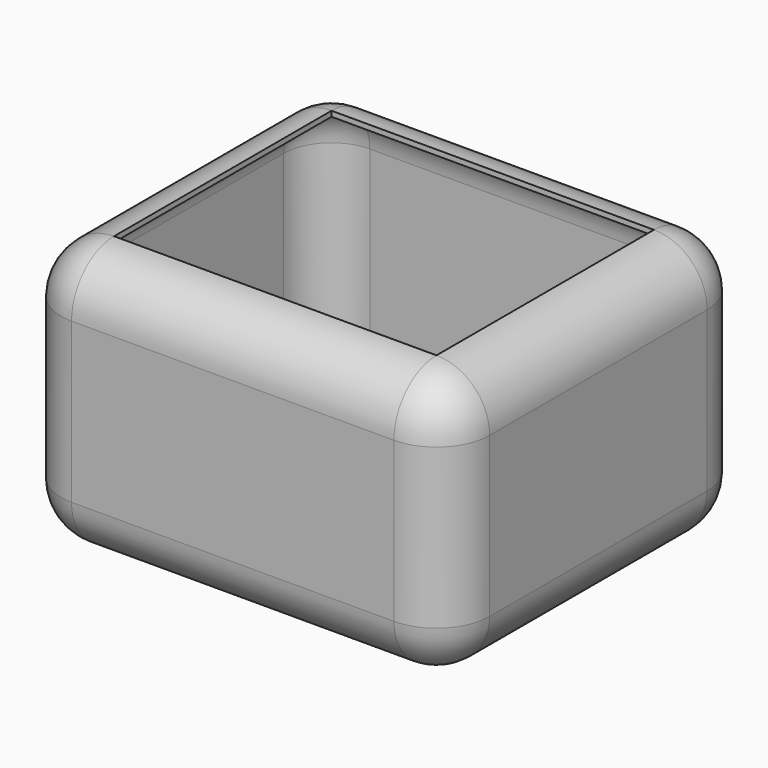
from build123d import *

# Parameters (mm, degrees)
F0_W     = 204.8915475607
F0_H     = 180.7192862034
F1_DEPTH = 127
F2_R     = 25.4
F3_T     = -2.54


# Not quite as in the source:
# - a shell that OpenCascade refuses in one call is made with other operations: the cavity is built on its own and cut out


with BuildPart() as f1:
    # F0 (on Top) → F1 (new body)
    with BuildSketch(Plane.XY):
        Rectangle(F0_W, F0_H)
    extrude(amount=F1_DEPTH)

    # F2
    f2_edges = [f1.edges().sort_by_distance(p)[0] for p in [
        (-102.445774, -90.359643, 63.5),
        (102.445774, -90.359643, 63.5),
        (0, -90.359643, 0),
        (0, -90.359643, 127),
        (102.445774, 90.359643, 63.5),
        (102.445774, 0, 0),
        (102.445774, 0, 127),
        (0, 90.359643, 127),
        (-102.445774, 0, 127),
        (-102.445774, 90.359643, 63.5),
        (-102.445774, 0, 0),
        (0, 90.359643, 0),
    ]]
    fillet(f2_edges, radius=F2_R)

    # F3: a shell. OpenCascade refuses it in one call, so the cavity is built on its own and cut out:
    # the body offset inwards by the wall thickness, plus a prism from it out through each open face.
    f3_core = offset(f1.part, amount=F3_T, mode=Mode.PRIVATE)
    f3_exits = [f3_core.faces().sort_by_distance(p)[0] for p in [
        (0, 0, 124.46),
    ]]
    add(f3_core, mode=Mode.SUBTRACT)
    extrude(f3_exits, amount=-F3_T, mode=Mode.SUBTRACT)


solid = f1.part
